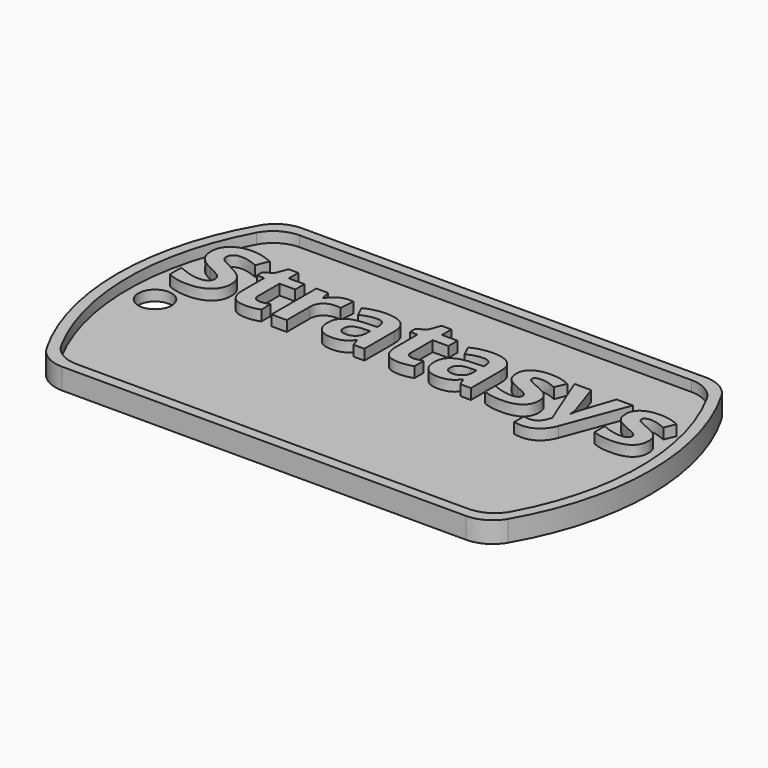
from build123d import *

# Parameters (mm, degrees)
F1_DEPTH     = 1
F3_DEPTH     = 1
F4_R         = 1.5875
F5_DEPTH     = 1
F6_TEXT_SIZE = 9.780972808
F7_DEPTH     = 1


# Not quite as in the source:
# - Text() gives the source's letters only with a copy of the font that has no kerning and outlines rounded to 1/6400 em; it was checked with that copy


with BuildPart() as f1:
    # F0 (on Top) → F1 (new body)
    with BuildSketch(Plane.XY):
        with BuildLine():
            ThreePointArc((-19.2474145991, 14.2875), (-20.8349145991, 13.862130657), (-21.9970452561, 12.7))
            ThreePointArc((-21.9970452561, 12.7), (-25.4, 0), (-21.9970452561, -12.7))
            ThreePointArc((-21.9970452561, -12.7), (-20.8349145991, -13.862130657), (-19.2474145991, -14.2875))
            Line((-19.2474145991, -14.2875), (19.2474145991, -14.2875))
            ThreePointArc((19.2474145991, -14.2875), (20.8349145991, -13.862130657), (21.9970452561, -12.7))
            ThreePointArc((21.9970452561, -12.7), (25.4, 0), (21.9970452561, 12.7))
            ThreePointArc((21.9970452561, 12.7), (20.8349145991, 13.862130657), (19.2474145991, 14.2875))
            Line((19.2474145991, 14.2875), (-19.2474145991, 14.2875))
        make_face()
    extrude(amount=F1_DEPTH)

    # F2 (on face) → F3 (join)
    with BuildSketch(Plane.XY.offset(1)):
        with BuildLine():
            Line((19.2474145991, 14.2875), (-19.2474145991, 14.2875))
            ThreePointArc((-19.2474145991, 14.2875), (-20.8349145991, 13.862130657), (-21.9970452561, 12.7))
            ThreePointArc((-21.9970452561, 12.7), (-25.4, 0), (-21.9970452561, -12.7))
            ThreePointArc((-21.9970452561, -12.7), (-20.8349145991, -13.862130657), (-19.2474145991, -14.2875))
            Line((-19.2474145991, -14.2875), (19.2474145991, -14.2875))
            ThreePointArc((19.2474145991, -14.2875), (20.8349145991, -13.862130657), (21.9970452561, -12.7))
            ThreePointArc((21.9970452561, -12.7), (25.4, 0), (21.9970452561, 12.7))
            ThreePointArc((21.9970452561, 12.7), (20.8349145991, 13.862130657), (19.2474145991, 14.2875))
        make_face()
        with BuildLine():
            ThreePointArc((-21.4526124879, 11.6252061249), (-20.2856017842, 12.8404540819), (-18.6611352482, 13.2875))
            Line((-18.6611352482, 13.2875), (18.6611352482, 13.2875))
            ThreePointArc((18.6611352482, 13.2875), (20.2856017842, 12.8404540819), (21.4526124879, 11.6252061249))
            ThreePointArc((21.4526124879, 11.6252061249), (24.4, 0), (21.4526124879, -11.6252061249))
            ThreePointArc((21.4526124879, -11.6252061249), (20.2856017842, -12.8404540819), (18.6611352482, -13.2875))
            Line((18.6611352482, -13.2875), (-18.6611352482, -13.2875))
            ThreePointArc((-18.6611352482, -13.2875), (-20.2856017842, -12.8404540819), (-21.4526124879, -11.6252061249))
            ThreePointArc((-21.4526124879, -11.6252061249), (-24.4, 0), (-21.4526124879, 11.6252061249))
        make_face(mode=Mode.SUBTRACT)
    extrude(amount=F3_DEPTH)

    # F4 (on face) → F5 (cut)
    with BuildSketch(Plane.XY.offset(1)):
        with Locations((-21.821282804, 0)):
            Circle(F4_R)
    extrude(amount=-F5_DEPTH, mode=Mode.SUBTRACT)

    # F6 (on face) → F7 (join)
    with BuildSketch(Plane.XY.offset(1)):
        with Locations((-22.7375791874, 2.0266924985)):
            Text('Stratasys', F6_TEXT_SIZE, font='Open Sans', font_style=FontStyle.BOLD, text_align=(TextAlign.LEFT, TextAlign.BOTTOM))
    extrude(amount=F7_DEPTH)


solid = f1.part
